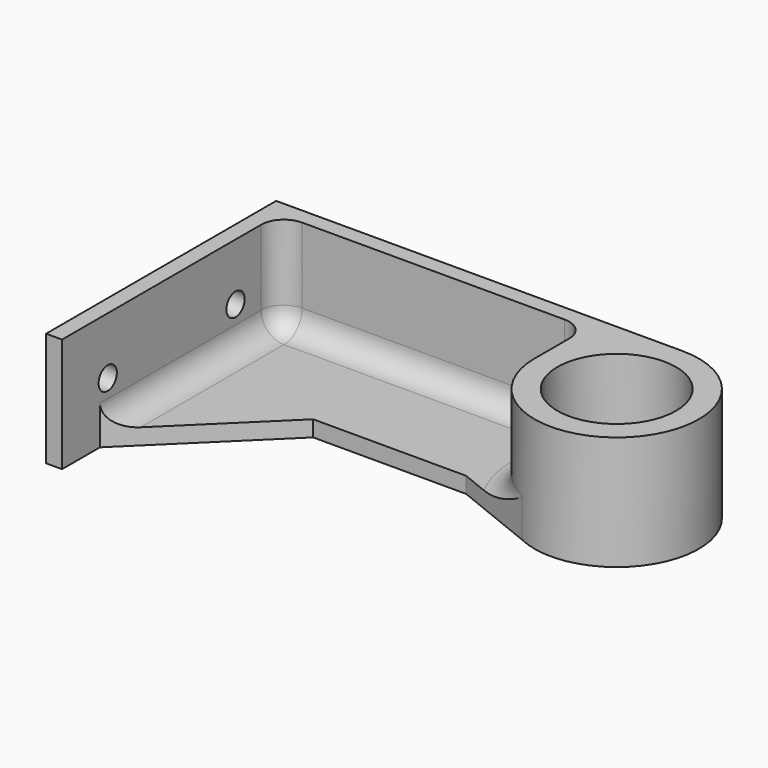
from build123d import *

# Parameters (mm, degrees)
F0_R      = 13
F1_DEPTH  = 25
F2_R      = 13
F3_DEPTH  = 3
F4_R      = 2.5
F5_DEPTH  = 25
F0_R_2    = 3
F6_DEPTH  = 30
F8_DEPTH  = 25
F9_DEPTH  = 3.5
F10_DEPTH = 30
F11_R     = 5


# Not quite as in the source:
# - a feature names something its author has since deleted; it is built from what else it names


with BuildPart() as f1:
    # F0 (on Top) → F1 (new body)
    with BuildSketch(Plane.XY):
        with BuildLine():
            Line((-44.2576195002, 24.5322410017), (-44.2576195002, -25.4677589983))
            Line((-44.2576195002, -25.4677589983), (-40.7576195002, -25.4677589983))
            Line((-40.7576195002, -25.4677589983), (-40.7576195002, 34.0321085225))
            Line((-40.7576195002, 34.0321085225), (26.7423804998, 34.0321085225))
            Line((26.7423804998, 34.0321085225), (26.7423804998, 19.5322410017))
            ThreePointArc((26.7423804998, 19.5322410017), (57.445862821, 6.7799260387), (44.8114401571, 37.5321085225))
            Line((44.8114401571, 37.5321085225), (44.6733208426, 37.5321085225))
            Line((44.6733208426, 37.5321085225), (-44.2576195002, 37.5321085225))
            Line((-44.2576195002, 37.5321085225), (-44.2576195002, 24.5322410017))
        make_face()
        with Locations((44.7423804998, 19.5322410017)):
            Circle(F0_R, mode=Mode.SUBTRACT)
    extrude(amount=F1_DEPTH)

    # F2 (on face) → F3 (join)
    with BuildSketch(Plane.XY.offset(25)):
        with BuildLine():
            ThreePointArc((26.7423804998, 19.5322410017), (29.5038185973, 9.9517279079), (36.9408506267, 3.3107696863))
            ThreePointArc((36.9408506267, 3.3107696863), (62.2844095115, 15.4977375434), (44.8114401571, 37.5321085225))
            Line((44.8114401571, 37.5321085225), (-44.2576195002, 37.5321085225))
            Line((-44.2576195002, 37.5321085225), (-44.2576195002, -25.4677589983))
            Line((-44.2576195002, -25.4677589983), (-40.7576195002, -25.4677589983))
            Line((-40.7576195002, -25.4677589983), (-40.7576195002, -15.0916781276))
            Line((-40.7576195002, -15.0916781276), (-40.7576195002, 34.0321085225))
            Line((-40.7576195002, 34.0321085225), (26.7423804998, 34.0321085225))
            Line((26.7423804998, 34.0321085225), (26.7423804998, 19.5322410017))
        make_face()
        with Locations((44.7423804998, 19.5322410017)):
            Circle(F2_R, mode=Mode.SUBTRACT)
    extrude(amount=-F3_DEPTH)

    # F4 (on face) → F5 (cut)
    with BuildSketch(Plane(origin=(-44.2576195002, 0, 0), x_dir=(0, -1, 0), z_dir=(-1, 0, 0))):
        with Locations((12.9677589983, 12.5)):
            Circle(F4_R)
    extrude(amount=-F5_DEPTH, mode=Mode.SUBTRACT)

    # F0 (on Top) → F6 (cut)
    with BuildSketch(Plane.XY):
        with Locations((44.7423804998, 19.5322410017)):
            Circle(F0_R_2)
    extrude(amount=F6_DEPTH, mode=Mode.SUBTRACT)

    # F4 (on face) → F8 (cut)
    with BuildSketch(Plane(origin=(-44.2576195002, 0, 0), x_dir=(0, -1, 0), z_dir=(-1, 0, 0))):
        with Locations((-22.0322410017, 12.5)):
            Circle(F4_R)
    extrude(amount=-F8_DEPTH, mode=Mode.SUBTRACT)

    # F2 (on face) → F9 (join)
    with BuildSketch(Plane.XY.offset(25)):
        with BuildLine():
            Line((18.9116307646, 10.5619383976), (36.9408506267, 3.3107696863))
            ThreePointArc((36.9408506267, 3.3107696863), (29.5038185973, 9.9517279079), (26.7423804998, 19.5322410017))
            Line((26.7423804998, 19.5322410017), (26.7423804998, 34.0321085225))
            Line((26.7423804998, 34.0321085225), (-40.7576195002, 34.0321085225))
            Line((-40.7576195002, 34.0321085225), (-40.7576195002, -15.0916781276))
            Line((-40.7576195002, -15.0916781276), (-14.5708816946, 10.5619383976))
            Line((-14.5708816946, 10.5619383976), (18.9116307646, 10.5619383976))
        make_face()
        with Locations((44.7423804998, 19.5322410017)):
            Circle(F2_R)
    extrude(amount=-F9_DEPTH)

    # F0 (on Top) → F10 (cut)
    with BuildSketch(Plane.XY):
        with Locations((44.7423804998, 19.5322410017)):
            Circle(F0_R_2)
    extrude(amount=F10_DEPTH, mode=Mode.SUBTRACT)

    # F11
    f11_edges = [f1.edges().sort_by_distance(p)[0] for p in [
        (26.74238, 34.032109, 10.75),
        (26.74238, 26.782175, 21.5),
        (-7.00762, 34.032109, 21.5),
        (-40.75762, 34.032109, 10.75),
        (-40.75762, 9.470215, 21.5),
    ]]
    fillet(f11_edges, radius=F11_R)


with BuildPart() as f13_1:
    # F13: instance of F1
    add(f1.part.mirror(Plane.XY.offset(50)))


solid = f13_1.part
